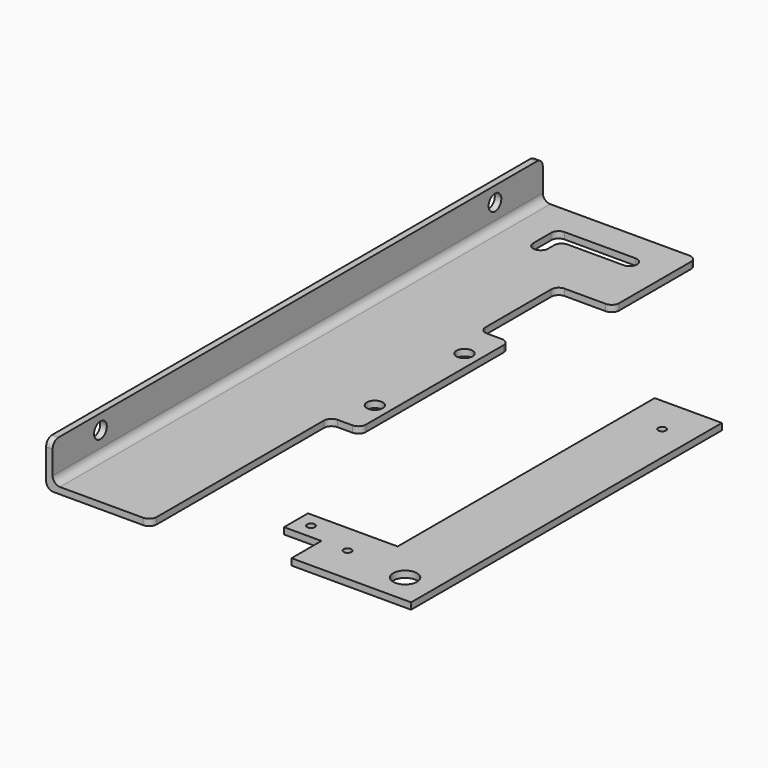
from build123d import *

# Parameters (mm, degrees)
F1_DEPTH  = 19.05
F2_DEPTH  = 2.778125
F3_T      = -2.778125
F5_DEPTH  = 25.4
F7_D      = 6.7564
F7_DEPTH  = 12.7
F7_TIP    = 2.0298273432
F9_D      = 3.2639
F9_DEPTH  = 12.7
F9_TIP    = 0.9805744872
F12_D     = 6.7564
F12_DEPTH = 12.7
F12_TIP   = 2.0298273432
F13_R     = 3.17499
F14_D     = 10.0838
F14_DEPTH = 12.7
F14_TIP   = 3.0294791551


# Not quite as in the source:
# - a fillet or chamfer is up to 0.001 mm smaller than in the source, because OpenCascade refuses the exact size
# - a feature names something its author has since deleted; it is built from what else it names


with BuildPart() as f1:
    # F0 (on Top) → F1 (new body)
    with BuildSketch(Plane.XY):
        Polygon((24.9401164524, 198.6622305675), (-43.3223835476, 198.6622305675), (-43.3223835476, -61.6877694325), (1.1276164524, -61.6877694325), (1.1276164524, 33.5622305675), (13.8276164524, 33.5622305675), (13.8276164524, 112.9372305675), (1.1276164524, 112.9372305675), (1.1276164524, 154.2122305675), (24.9401164524, 154.2122305675), align=None)
    extrude(amount=F1_DEPTH)

    # F3
    f3_openings = [f1.faces().sort_by_distance(p)[0] for p in [
        (-16.336644, 77.216721, 19.05),
        (13.827616, 73.249731, 9.525),
        (24.940116, 176.437231, 9.525),
        (-21.097384, -61.687769, 9.525),
        (1.127616, -14.062769, 9.525),
        (7.477616, 33.562231, 9.525),
        (7.477616, 112.937231, 9.525),
        (1.127616, 133.574731, 9.525),
        (13.033866, 154.212231, 9.525),
        (-9.191134, 198.662231, 9.525),
    ]]
    offset(amount=F3_T, openings=f3_openings)

    # F4 (on face) → F5 (cut)
    with BuildSketch(Plane.XY.offset(2.778125)):
        Polygon((12.2401164524, 179.6122305675), (12.2401164524, 185.9622305675), (-24.2723835476, 185.9622305675), (-24.2723835476, 170.0872305675), (-17.9223835476, 170.0872305675), (-17.9223835476, 179.6122305675), align=None)
    extrude(amount=-F5_DEPTH, mode=Mode.SUBTRACT)

    # F7
    with Locations(Plane.XY.offset(2.778125)):
        with Locations((7.4776164524, 97.0622305675), (7.4776164524, 49.4372305675)):
            Hole(F7_D / 2, depth=F7_DEPTH)
            with Locations((0, 0, -(F7_DEPTH + F7_TIP / 2))):  # 118° drill point
                Cone(0, F7_D / 2, F7_TIP, mode=Mode.SUBTRACT)

    # F12
    with Locations(Plane.YZ.offset(-40.5442585476)):
        with Locations((-36.2877694325, 12.7), (173.2622305675, 12.7)):
            Hole(F12_D / 2, depth=F12_DEPTH)
            with Locations((0, 0, -(F12_DEPTH + F12_TIP / 2))):  # 118° drill point
                Cone(0, F12_D / 2, F12_TIP, mode=Mode.SUBTRACT)

    # F13 (radius 3.175 in the source; OpenCascade refuses exactly that, so slightly less here)
    f13_edges = [f1.edges().sort_by_distance(p)[0] for p in [
        (-24.272384, 170.087231, 1.389063),
        (-24.272384, 185.962231, 1.389063),
        (-17.922384, 170.087231, 1.389063),
        (-17.922384, 179.612231, 1.389063),
        (12.240116, 185.962231, 1.389063),
        (12.240116, 179.612231, 1.389063),
        (24.940116, 198.662231, 1.389063),
        (1.127616, 112.937231, 1.389063),
        (1.127616, 154.212231, 1.389063),
        (24.940116, 154.212231, 1.389063),
        (13.827616, 112.937231, 1.389063),
        (13.827616, 33.562231, 1.389063),
        (1.127616, 33.562231, 1.389063),
        (1.127616, -61.687769, 1.389063),
        (-40.544259, 68.487231, 2.778125),
        (-41.933321, -61.687769, 19.05),
        (-41.933321, 198.662231, 19.05),
        (-43.322384, 68.487231, 0),
    ]]
    fillet(f13_edges, radius=F13_R)


with BuildPart() as f2:
    # F0 (on Top) → F2 (new body)
    with BuildSketch(Plane.XY):
        Polygon((105.3239927769, -53.6233703196), (105.3239927769, 111.4766296804), (76.7489927769, 111.4766296804), (76.7489927769, -25.0483703196), (38.6489927769, -25.0483703196), (38.6489927769, -37.7483703196), (54.5239927769, -37.7483703196), (54.5239927769, -53.6233703196), align=None)
    extrude(amount=F2_DEPTH)

    # F9
    with Locations(Plane(origin=(0, 0, 0), x_dir=(1, 0, 0), z_dir=(0, 0, -1))):
        with Locations((65.6364927769, 37.7483703196), (44.9989927769, 31.3983703196), (92.6239927769, -95.6016296804)):
            Hole(F9_D / 2, depth=F9_DEPTH)
            with Locations((0, 0, -(F9_DEPTH + F9_TIP / 2))):  # 118° drill point
                Cone(0, F9_D / 2, F9_TIP, mode=Mode.SUBTRACT)

    # F14
    with Locations(Plane(origin=(0, 0, 0), x_dir=(1, 0, 0), z_dir=(0, 0, -1))):
        with Locations((92.6239927769, 40.9233703196)):
            Hole(F14_D / 2, depth=F14_DEPTH)
            with Locations((0, 0, -(F14_DEPTH + F14_TIP / 2))):  # 118° drill point
                Cone(0, F14_D / 2, F14_TIP, mode=Mode.SUBTRACT)


solid = Compound([f1.part, f2.part])
